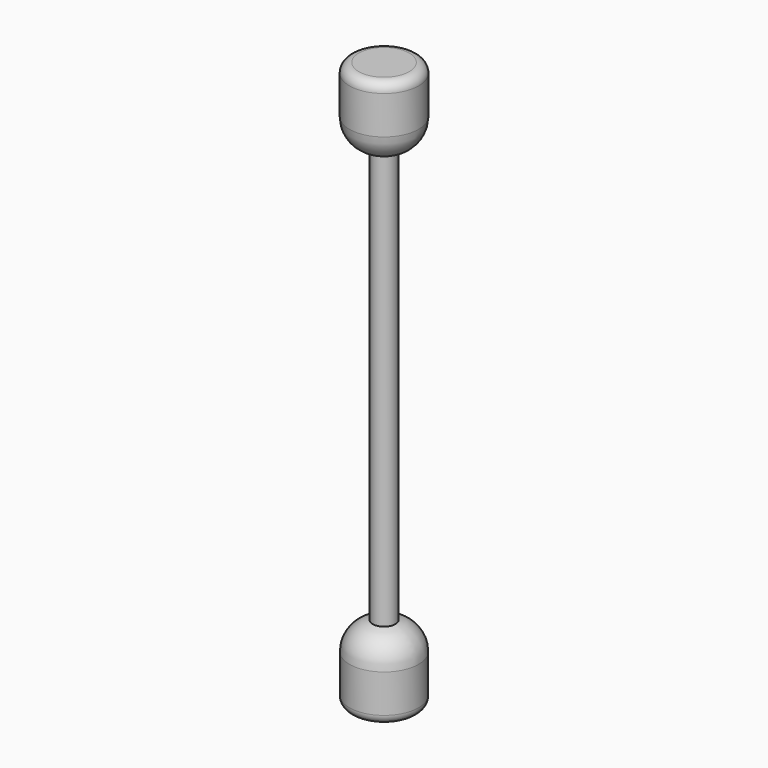
from build123d import *

# Parameters (mm, degrees)
F0_R     = 9.1524845949
F1_DEPTH = 20
F2_R     = 3.008201979
F3_DEPTH = 110
F4_R     = 9.1770067028
F5_DEPTH = 20
F7_R     = 2.5


# Not quite as in the source:
# - a fillet or chamfer that OpenCascade refuses, or shapes differently, is made with other operations: its cross-section is extruded or revolved along the edge and cut away or added


with BuildPart() as f1:
    # F0 (on Top) → F1 (new body)
    with BuildSketch(Plane.XY):
        Circle(F0_R)
    extrude(amount=F1_DEPTH)

    # F2 (on face) → F3 (join)
    with BuildSketch(Plane.XY.offset(20)):
        Circle(F2_R)
    extrude(amount=F3_DEPTH)

    # F4 (on face) → F5 (join)
    with BuildSketch(Plane.XY.offset(130)):
        Circle(F4_R)
    extrude(amount=F5_DEPTH)

    # F6: fillet of radius 7.5 on 2 edges, made by hand

    # F6_s1 → F6_t2 (revolve, cut)
    with BuildSketch(Plane.XZ):
        with BuildLine():
            ThreePointArc((3.008201979, 20), (7.4152044554, 17.4236593265), (9.1524845949, 12.6235489309))
            Line((9.1524845949, 12.6235489309), (9.1524845949, 20))
            Line((9.1524845949, 20), (3.008201979, 20))
        make_face()
    revolve(axis=Axis((0, 0, 20), (0, 0, 1)), mode=Mode.SUBTRACT)

    # F6_s3 → F6_t4 (revolve, cut)
    with BuildSketch(Plane.XZ):
        with BuildLine():
            ThreePointArc((9.1770067028, 137.3809158738), (7.4317423427, 132.5712362884), (3.008201979, 130))
            Line((3.008201979, 130), (9.1770067028, 130))
            Line((9.1770067028, 130), (9.1770067028, 137.3809158738))
        make_face()
    revolve(axis=Axis((0, 0, 130), (0, 0, 1)), mode=Mode.SUBTRACT)

    # F7
    f7_edges = [f1.edges().sort_by_distance(p)[0] for p in [
        (-9.177007, 0, 150),
        (-9.152485, 0, 0),
    ]]
    fillet(f7_edges, radius=F7_R)


solid = f1.part
